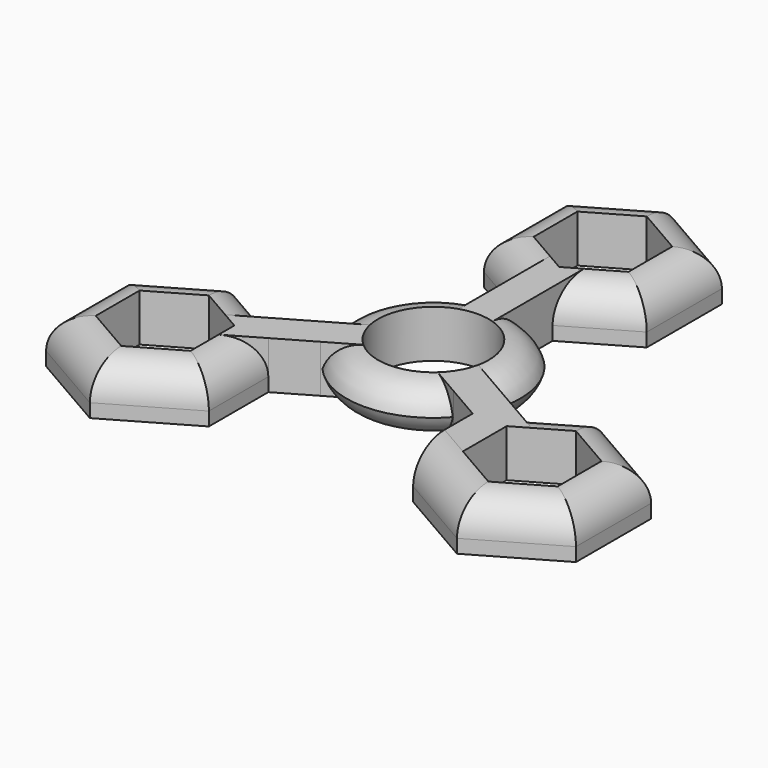
from build123d import *

# Parameters (mm, degrees)
F0_R          = 8.15
F1_DEPTH      = 7
F2_T4_DEPTH   = 35.9367513459
F2_T10_DEPTH  = 38.8235026919
F2_T16_DEPTH  = 38.8235026919
F2_T22_DEPTH  = 38.8235026919
F2_T28_DEPTH  = 38.8235026919
F2_T34_DEPTH  = 35.9367513459
F2_T40_DEPTH  = 38.8235026919
F2_T46_DEPTH  = 38.8235026919
F2_T52_DEPTH  = 38.8235026919
F2_T58_DEPTH  = 35.9367513459
F2_T64_DEPTH  = 38.8235026919
F2_T70_DEPTH  = 38.8235026919
F2_T76_DEPTH  = 38.8235026919
F2_T82_DEPTH  = 38.8235026919
F2_T88_DEPTH  = 38.8235026919
F2_T94_DEPTH  = 35.9367513459
F2_T100_DEPTH = 35.9367513459
F2_T106_ANGLE = 208.0615087698
F2_T112_ANGLE = 208.0615087698
F2_T118_ANGLE = 208.0615087698
F2_T124_ANGLE = 208.0615087698
F2_T130_ANGLE = 208.0615087698
F2_T136_ANGLE = 208.0615087698
F2_T143_DEPTH = 35.9367513459
F2_T147_DEPTH = 38.8235026919
F2_T154_DEPTH = 38.8235026919
F2_T158_DEPTH = 38.8235026919
F2_T165_DEPTH = 38.8235026919
F2_T169_DEPTH = 38.8235026919
F2_T176_DEPTH = 38.8235026919
F2_T180_DEPTH = 38.8235026919
F2_T187_DEPTH = 38.8235026919
F2_T191_DEPTH = 35.9367513459
F2_T198_DEPTH = 38.8235026919
F2_T202_DEPTH = 38.8235026919
F2_T209_DEPTH = 38.8235026919
F2_T213_DEPTH = 38.8235026919
F2_T220_DEPTH = 38.8235026919
F2_T224_DEPTH = 38.8235026919
F2_T231_DEPTH = 38.8235026919
F2_T235_DEPTH = 35.9367513459
F2_T242_DEPTH = 38.8235026919
F2_T246_DEPTH = 38.8235026919
F2_T253_DEPTH = 38.8235026919
F2_T257_DEPTH = 35.9367513459
F2_T264_DEPTH = 38.8235026919
F2_T268_DEPTH = 38.8235026919
F2_T275_DEPTH = 38.8235026919
F2_T279_DEPTH = 38.8235026919
F2_T286_DEPTH = 35.9367513459
F2_T290_DEPTH = 38.8235026919


# Not quite as in the source:
# - a fillet or chamfer that OpenCascade refuses, or shapes differently, is made with other operations: its cross-section is extruded or revolved along the edge and cut away or added


with BuildPart() as f1:
    # F0 (on Top) → F1 (new body)
    with BuildSketch(Plane.XY):
        with BuildLine():
            ThreePointArc((12.298189897, -4.2136119016), (12.8233472358, -2.1358290357), (13, 0))
            ThreePointArc((13, 0), (10.0374299499, 8.2613558209), (2.5, 12.7573508222))
            ThreePointArc((2.5, 12.7573508222), (0, 13), (-2.5, 12.7573508222))
            ThreePointArc((-2.5, 12.7573508222), (-11.2583302492, 6.5), (-12.298189897, -4.2136119016))
            ThreePointArc((-12.298189897, -4.2136119016), (-11.2583302492, -6.5), (-9.798189897, -8.5437389205))
            ThreePointArc((-9.798189897, -8.5437389205), (0, -13), (9.798189897, -8.5437389205))
            ThreePointArc((9.798189897, -8.5437389205), (11.2583302492, -6.5), (12.298189897, -4.2136119016))
        make_face()
        Circle(F0_R, mode=Mode.SUBTRACT)
        with BuildLine():
            ThreePointArc((-2.5, 12.7573508222), (0, 13), (2.5, 12.7573508222))
            Line((2.5, 12.7573508222), (2.5, 18.7963702892))
            Line((2.5, 18.7963702892), (11.9715045005, 24.2647459622))
            Line((11.9715045005, 24.2647459622), (11.9715045005, 38.0882486541))
            Line((11.9715045005, 38.0882486541), (0, 45))
            Line((0, 45), (-11.9715045005, 38.0882486541))
            Line((-11.9715045005, 38.0882486541), (-11.9715045005, 24.2647459622))
            Line((-11.9715045005, 24.2647459622), (-5.9857522502, 20.8088702892))
            Line((-5.9857522502, 20.8088702892), (-2.5, 18.7963702892))
            Line((-2.5, 18.7963702892), (-2.5, 12.7573508222))
        make_face()
        Polygon((0, 39.2264973081), (6.9715045005, 35.2014973081), (6.9715045005, 27.1514973081), (0, 23.1264973081), (-6.9715045005, 27.1514973081), (-6.9715045005, 35.2014973081), align=None, mode=Mode.SUBTRACT)
        with BuildLine():
            Line((17.5281341694, -7.2331216351), (12.298189897, -4.2136119016))
            ThreePointArc((12.298189897, -4.2136119016), (11.2583302492, -6.5), (9.798189897, -8.5437389205))
            Line((9.798189897, -8.5437389205), (15.0281341694, -11.5632486541))
            Line((15.0281341694, -11.5632486541), (15.0281341694, -22.5))
            Line((15.0281341694, -22.5), (26.9996386698, -29.4117513459))
            Line((26.9996386698, -29.4117513459), (38.9711431703, -22.5))
            Line((38.9711431703, -22.5), (38.9711431703, -8.6764973081))
            Line((38.9711431703, -8.6764973081), (26.9996386698, -1.7647459622))
            Line((26.9996386698, -1.7647459622), (21.0138864196, -5.2206216351))
            Line((21.0138864196, -5.2206216351), (17.5281341694, -7.2331216351))
        make_face()
        Polygon((33.9711431703, -19.6132486541), (26.9996386698, -23.6382486541), (20.0281341694, -19.6132486541), (20.0281341694, -11.5632486541), (26.9996386698, -7.5382486541), (33.9711431703, -11.5632486541), align=None, mode=Mode.SUBTRACT)
        with BuildLine():
            ThreePointArc((-9.798189897, -8.5437389205), (-11.2583302492, -6.5), (-12.298189897, -4.2136119016))
            Line((-12.298189897, -4.2136119016), (-17.5281341694, -7.2331216351))
            Line((-17.5281341694, -7.2331216351), (-26.9996386698, -1.7647459622))
            Line((-26.9996386698, -1.7647459622), (-38.9711431703, -8.6764973081))
            Line((-38.9711431703, -8.6764973081), (-38.9711431703, -22.5))
            Line((-38.9711431703, -22.5), (-26.9996386698, -29.4117513459))
            Line((-26.9996386698, -29.4117513459), (-15.0281341694, -22.5))
            Line((-15.0281341694, -22.5), (-15.0281341694, -15.5882486541))
            Line((-15.0281341694, -15.5882486541), (-15.0281341694, -11.5632486541))
            Line((-15.0281341694, -11.5632486541), (-9.798189897, -8.5437389205))
        make_face()
        Polygon((-33.9711431703, -19.6132486541), (-33.9711431703, -11.5632486541), (-26.9996386698, -7.5382486541), (-20.0281341694, -11.5632486541), (-20.0281341694, -19.6132486541), (-26.9996386698, -23.6382486541), align=None, mode=Mode.SUBTRACT)
    extrude(amount=F1_DEPTH)

    # F2: fillet of radius 5 on 23 edges, made by hand


with BuildPart() as f2_tool2:
    # F2_s3 → F2_t4 (new body)
    with BuildSketch(Plane(origin=(0.8112504626, -0.468375673, 0), x_dir=(0, 0, 1), z_dir=(-0.8660254038, 0.5, 0))):
        with BuildLine():
            ThreePointArc((2, -15.0281341694), (5.5355339059, -16.4926002634), (7, -20.0281341694))
            Line((7, -20.0281341694), (7.1, -20.0281341694))
            Line((7.1, -20.0281341694), (7.1, -14.9281341694))
            Line((7.1, -14.9281341694), (2, -14.9281341694))
            Line((2, -14.9281341694), (2, -15.0281341694))
        make_face()
    extrude(amount=F2_T4_DEPTH)

    split(bisect_by=Plane(origin=(-1.25, 2.1650635095, 0), x_dir=(0, 0, 1), z_dir=(-0.5, 0.8660254038, 0)), keep=Keep.TOP)

    split(bisect_by=Plane(origin=(-5.9857522502, 10.3676270189, 0), x_dir=(0, 0, 1), z_dir=(0.5, -0.8660254038, 0)), keep=Keep.TOP)


with BuildPart() as f1_1:
    add(f1.part)

    # F2_t1: cut F2_tool2
    add(f2_tool2.part, mode=Mode.SUBTRACT)


with BuildPart() as f2_tool8:
    # F2_s9 → F2_t10 (new body)
    with BuildSketch(Plane(origin=(-10.1885688723, -5.8823729811, 0), x_dir=(0, 0, 1), z_dir=(-0.8660254038, -0.5, 0))):
        with BuildLine():
            ThreePointArc((2, 11.9715045005), (5.5355339059, 10.5070384064), (7, 6.9715045005))
            Line((7, 6.9715045005), (7.1, 6.9715045005))
            Line((7.1, 6.9715045005), (7.1, 12.0715045005))
            Line((7.1, 12.0715045005), (2, 12.0715045005))
            Line((2, 12.0715045005), (2, 11.9715045005))
        make_face()
    extrude(amount=F2_T10_DEPTH)

    split(bisect_by=Plane(origin=(-7.5140670847, -13.0147459622, 0), x_dir=(0, 0, 1), z_dir=(-0.5, -0.8660254038, 0)), keep=Keep.TOP)

    split(bisect_by=Plane.YZ.offset(-38.9711431703), keep=Keep.TOP)


with BuildPart() as f1_2:
    add(f1_1.part)

    # F2_t7: cut F2_tool8
    add(f2_tool8.part, mode=Mode.SUBTRACT)


with BuildPart() as f2_tool14:
    # F2_s15 → F2_t16 (new body)
    with BuildSketch(Plane.XZ.offset(-3.8235026919)):
        with BuildLine():
            ThreePointArc((-38.9711431703, 2), (-37.5066770762, 5.5355339059), (-33.9711431703, 7))
            Line((-33.9711431703, 7), (-33.9711431703, 7.1))
            Line((-33.9711431703, 7.1), (-39.0711431703, 7.1))
            Line((-39.0711431703, 7.1), (-39.0711431703, 2))
            Line((-39.0711431703, 2), (-38.9711431703, 2))
        make_face()
    extrude(amount=F2_T16_DEPTH)

    split(bisect_by=Plane(origin=(-5.9857522502, 10.3676270189, 0), x_dir=(0, 0, 1), z_dir=(0.5, -0.8660254038, 0)), keep=Keep.TOP)

    split(bisect_by=Plane(origin=(-19.4855715851, -33.75, 0), x_dir=(0, 0, 1), z_dir=(0.5, 0.8660254038, 0)), keep=Keep.TOP)


with BuildPart() as f1_3:
    add(f1_2.part)

    # F2_t13: cut F2_tool14
    add(f2_tool14.part, mode=Mode.SUBTRACT)


with BuildPart() as f2_tool20:
    # F2_s21 → F2_t22 (new body)
    with BuildSketch(Plane(origin=(-30.3108891325, 17.5, 0), x_dir=(0, 0, 1), z_dir=(0.8660254038, -0.5, 0))):
        with BuildLine():
            ThreePointArc((2, 38.9711431703), (5.5355339059, 37.5066770762), (7, 33.9711431703))
            Line((7, 33.9711431703), (7.1, 33.9711431703))
            Line((7.1, 33.9711431703), (7.1, 39.0711431703))
            Line((7.1, 39.0711431703), (2, 39.0711431703))
            Line((2, 39.0711431703), (2, 38.9711431703))
        make_face()
    extrude(amount=F2_T22_DEPTH)

    split(bisect_by=Plane.YZ.offset(-38.9711431703), keep=Keep.TOP)

    split(bisect_by=Plane(origin=(5.9857522502, -10.3676270189, 0), x_dir=(0, 0, 1), z_dir=(-0.5, 0.8660254038, 0)), keep=Keep.TOP)


with BuildPart() as f1_4:
    add(f1_3.part)

    # F2_t19: cut F2_tool20
    add(f2_tool20.part, mode=Mode.SUBTRACT)


with BuildPart() as f2_tool26:
    # F2_s27 → F2_t28 (new body)
    with BuildSketch(Plane(origin=(-43.8107084674, -25.294124327, 0), x_dir=(0, 0, 1), z_dir=(0.8660254038, 0.5, 0))):
        with BuildLine():
            ThreePointArc((2, 11.9715045005), (5.5355339059, 10.5070384064), (7, 6.9715045005))
            Line((7, 6.9715045005), (7.1, 6.9715045005))
            Line((7.1, 6.9715045005), (7.1, 12.0715045005))
            Line((7.1, 12.0715045005), (2, 12.0715045005))
            Line((2, 12.0715045005), (2, 11.9715045005))
        make_face()
    extrude(amount=F2_T28_DEPTH)

    split(bisect_by=Plane(origin=(-19.4855715851, -33.75, 0), x_dir=(0, 0, 1), z_dir=(0.5, 0.8660254038, 0)), keep=Keep.TOP)

    split(bisect_by=Plane.YZ.offset(-15.0281341694), keep=Keep.BOTTOM)


with BuildPart() as f1_5:
    add(f1_4.part)

    # F2_t25: cut F2_tool26
    add(f2_tool26.part, mode=Mode.SUBTRACT)


with BuildPart() as f2_tool32:
    # F2_s33 → F2_t34 (new body)
    with BuildSketch(Plane.XZ.offset(35)):
        with BuildLine():
            ThreePointArc((-15.0281341694, 2), (-16.4926002634, 5.5355339059), (-20.0281341694, 7))
            Line((-20.0281341694, 7), (-20.0281341694, 7.1))
            Line((-20.0281341694, 7.1), (-14.9281341694, 7.1))
            Line((-14.9281341694, 7.1), (-14.9281341694, 2))
            Line((-14.9281341694, 2), (-15.0281341694, 2))
        make_face()
    extrude(amount=-F2_T34_DEPTH)

    split(bisect_by=Plane(origin=(5.9857522502, -10.3676270189, 0), x_dir=(0, 0, 1), z_dir=(-0.5, 0.8660254038, 0)), keep=Keep.TOP)

    split(bisect_by=Plane(origin=(1.25, -2.1650635095, 0), x_dir=(0, 0, 1), z_dir=(0.5, -0.8660254038, 0)), keep=Keep.TOP)


with BuildPart() as f1_6:
    add(f1_5.part)

    # F2_t31: cut F2_tool32
    add(f2_tool32.part, mode=Mode.SUBTRACT)


with BuildPart() as f2_tool38:
    # F2_s39 → F2_t40 (new body)
    with BuildSketch(Plane(origin=(-3.3112504626, -1.9117513459, 0), x_dir=(0, 0, 1), z_dir=(0.8660254038, 0.5, 0))):
        with BuildLine():
            ThreePointArc((2, 38.9711431703), (5.5355339059, 37.5066770762), (7, 33.9711431703))
            Line((7, 33.9711431703), (7.1, 33.9711431703))
            Line((7.1, 33.9711431703), (7.1, 39.0711431703))
            Line((7.1, 39.0711431703), (2, 39.0711431703))
            Line((2, 39.0711431703), (2, 38.9711431703))
        make_face()
    extrude(amount=F2_T40_DEPTH)

    split(bisect_by=Plane(origin=(-5.9857522502, -10.3676270189, 0), x_dir=(0, 0, 1), z_dir=(0.5, 0.8660254038, 0)), keep=Keep.TOP)

    split(bisect_by=Plane.YZ.offset(38.9711431703), keep=Keep.BOTTOM)


with BuildPart() as f1_7:
    add(f1_6.part)

    # F2_t37: cut F2_tool38
    add(f2_tool38.part, mode=Mode.SUBTRACT)


with BuildPart() as f2_tool44:
    # F2_s45 → F2_t46 (new body)
    with BuildSketch(Plane.XZ.offset(35)):
        with BuildLine():
            ThreePointArc((38.9711431703, 2), (37.5066770762, 5.5355339059), (33.9711431703, 7))
            Line((33.9711431703, 7), (33.9711431703, 7.1))
            Line((33.9711431703, 7.1), (39.0711431703, 7.1))
            Line((39.0711431703, 7.1), (39.0711431703, 2))
            Line((39.0711431703, 2), (38.9711431703, 2))
        make_face()
    extrude(amount=-F2_T46_DEPTH)

    split(bisect_by=Plane(origin=(19.4855715851, -33.75, 0), x_dir=(0, 0, 1), z_dir=(-0.5, 0.8660254038, 0)), keep=Keep.TOP)

    split(bisect_by=Plane(origin=(5.9857522502, 10.3676270189, 0), x_dir=(0, 0, 1), z_dir=(-0.5, -0.8660254038, 0)), keep=Keep.TOP)


with BuildPart() as f1_8:
    add(f1_7.part)

    # F2_t43: cut F2_tool44
    add(f2_tool44.part, mode=Mode.SUBTRACT)


with BuildPart() as f2_tool50:
    # F2_s51 → F2_t52 (new body)
    with BuildSketch(Plane(origin=(43.8107084674, -25.294124327, 0), x_dir=(0, 0, 1), z_dir=(-0.8660254038, 0.5, 0))):
        with BuildLine():
            ThreePointArc((2, 11.9715045005), (5.5355339059, 10.5070384064), (7, 6.9715045005))
            Line((7, 6.9715045005), (7.1, 6.9715045005))
            Line((7.1, 6.9715045005), (7.1, 12.0715045005))
            Line((7.1, 12.0715045005), (2, 12.0715045005))
            Line((2, 12.0715045005), (2, 11.9715045005))
        make_face()
    extrude(amount=F2_T52_DEPTH)

    split(bisect_by=Plane.YZ.offset(38.9711431703), keep=Keep.BOTTOM)

    split(bisect_by=Plane(origin=(7.5140670847, -13.0147459622, 0), x_dir=(0, 0, 1), z_dir=(0.5, -0.8660254038, 0)), keep=Keep.TOP)


with BuildPart() as f1_9:
    add(f1_8.part)

    # F2_t49: cut F2_tool50
    add(f2_tool50.part, mode=Mode.SUBTRACT)


with BuildPart() as f2_tool56:
    # F2_s57 → F2_t58 (new body)
    with BuildSketch(Plane(origin=(30.3108891325, 17.5, 0), x_dir=(0, 0, 1), z_dir=(-0.8660254038, -0.5, 0))):
        with BuildLine():
            ThreePointArc((2, -15.0281341694), (5.5355339059, -16.4926002634), (7, -20.0281341694))
            Line((7, -20.0281341694), (7.1, -20.0281341694))
            Line((7.1, -20.0281341694), (7.1, -14.9281341694))
            Line((7.1, -14.9281341694), (2, -14.9281341694))
            Line((2, -14.9281341694), (2, -15.0281341694))
        make_face()
    extrude(amount=F2_T58_DEPTH)

    split(bisect_by=Plane(origin=(5.9857522502, 10.3676270189, 0), x_dir=(0, 0, 1), z_dir=(-0.5, -0.8660254038, 0)), keep=Keep.TOP)

    split(bisect_by=Plane(origin=(1.25, 2.1650635095, 0), x_dir=(0, 0, 1), z_dir=(0.5, 0.8660254038, 0)), keep=Keep.TOP)


with BuildPart() as f1_10:
    add(f1_9.part)

    # F2_t55: cut F2_tool56
    add(f2_tool56.part, mode=Mode.SUBTRACT)


with BuildPart() as f2_tool62:
    # F2_s63 → F2_t64 (new body)
    with BuildSketch(Plane(origin=(10.1885688723, -5.8823729811, 0), x_dir=(0, 0, 1), z_dir=(0.8660254038, -0.5, 0))):
        with BuildLine():
            ThreePointArc((2, 11.9715045005), (5.5355339059, 10.5070384064), (7, 6.9715045005))
            Line((7, 6.9715045005), (7.1, 6.9715045005))
            Line((7.1, 6.9715045005), (7.1, 12.0715045005))
            Line((7.1, 12.0715045005), (2, 12.0715045005))
            Line((2, 12.0715045005), (2, 11.9715045005))
        make_face()
    extrude(amount=F2_T64_DEPTH)

    split(bisect_by=Plane.YZ.offset(15.0281341694), keep=Keep.TOP)

    split(bisect_by=Plane(origin=(19.4855715851, -33.75, 0), x_dir=(0, 0, 1), z_dir=(-0.5, 0.8660254038, 0)), keep=Keep.TOP)


with BuildPart() as f1_11:
    add(f1_10.part)

    # F2_t61: cut F2_tool62
    add(f2_tool62.part, mode=Mode.SUBTRACT)


with BuildPart() as f2_tool68:
    # F2_s69 → F2_t70 (new body)
    with BuildSketch(Plane.XZ.offset(-50.5882486541)):
        with BuildLine():
            ThreePointArc((-11.9715045005, 2), (-10.5070384064, 5.5355339059), (-6.9715045005, 7))
            Line((-6.9715045005, 7), (-6.9715045005, 7.1))
            Line((-6.9715045005, 7.1), (-12.0715045005, 7.1))
            Line((-12.0715045005, 7.1), (-12.0715045005, 2))
            Line((-12.0715045005, 2), (-11.9715045005, 2))
        make_face()
    extrude(amount=F2_T70_DEPTH)

    split(bisect_by=Plane(origin=(-19.4855715851, 33.75, 0), x_dir=(0, 0, 1), z_dir=(0.5, -0.8660254038, 0)), keep=Keep.TOP)

    split(bisect_by=Plane(origin=(7.5140670847, 13.0147459622, 0), x_dir=(0, 0, 1), z_dir=(0.5, 0.8660254038, 0)), keep=Keep.TOP)


with BuildPart() as f1_12:
    add(f1_11.part)

    # F2_t67: cut F2_tool68
    add(f2_tool68.part, mode=Mode.SUBTRACT)


with BuildPart() as f2_tool74:
    # F2_s75 → F2_t76 (new body)
    with BuildSketch(Plane(origin=(30.3108891325, 17.5, 0), x_dir=(0, 0, 1), z_dir=(-0.8660254038, -0.5, 0))):
        with BuildLine():
            ThreePointArc((2, 38.9711431703), (5.5355339059, 37.5066770762), (7, 33.9711431703))
            Line((7, 33.9711431703), (7.1, 33.9711431703))
            Line((7.1, 33.9711431703), (7.1, 39.0711431703))
            Line((7.1, 39.0711431703), (2, 39.0711431703))
            Line((2, 39.0711431703), (2, 38.9711431703))
        make_face()
    extrude(amount=F2_T76_DEPTH)

    split(bisect_by=Plane(origin=(19.4855715851, 33.75, 0), x_dir=(0, 0, 1), z_dir=(-0.5, -0.8660254038, 0)), keep=Keep.TOP)

    split(bisect_by=Plane.YZ.offset(-11.9715045005), keep=Keep.TOP)


with BuildPart() as f1_13:
    add(f1_12.part)

    # F2_t73: cut F2_tool74
    add(f2_tool74.part, mode=Mode.SUBTRACT)


with BuildPart() as f2_tool80:
    # F2_s81 → F2_t82 (new body)
    with BuildSketch(Plane(origin=(3.3112504626, -1.9117513459, 0), x_dir=(0, 0, 1), z_dir=(-0.8660254038, 0.5, 0))):
        with BuildLine():
            ThreePointArc((2, 38.9711431703), (5.5355339059, 37.5066770762), (7, 33.9711431703))
            Line((7, 33.9711431703), (7.1, 33.9711431703))
            Line((7.1, 33.9711431703), (7.1, 39.0711431703))
            Line((7.1, 39.0711431703), (2, 39.0711431703))
            Line((2, 39.0711431703), (2, 38.9711431703))
        make_face()
    extrude(amount=F2_T82_DEPTH)

    split(bisect_by=Plane.YZ.offset(11.9715045005), keep=Keep.BOTTOM)

    split(bisect_by=Plane(origin=(-19.4855715851, 33.75, 0), x_dir=(0, 0, 1), z_dir=(0.5, -0.8660254038, 0)), keep=Keep.TOP)


with BuildPart() as f1_14:
    add(f1_13.part)

    # F2_t79: cut F2_tool80
    add(f2_tool80.part, mode=Mode.SUBTRACT)


with BuildPart() as f2_tool86:
    # F2_s87 → F2_t88 (new body)
    with BuildSketch(Plane.XZ.offset(-11.7647459622)):
        with BuildLine():
            ThreePointArc((11.9715045005, 2), (10.5070384064, 5.5355339059), (6.9715045005, 7))
            Line((6.9715045005, 7), (6.9715045005, 7.1))
            Line((6.9715045005, 7.1), (12.0715045005, 7.1))
            Line((12.0715045005, 7.1), (12.0715045005, 2))
            Line((12.0715045005, 2), (11.9715045005, 2))
        make_face()
    extrude(amount=-F2_T88_DEPTH)

    split(bisect_by=Plane(origin=(-7.5140670847, 13.0147459622, 0), x_dir=(0, 0, 1), z_dir=(-0.5, 0.8660254038, 0)), keep=Keep.TOP)

    split(bisect_by=Plane(origin=(19.4855715851, 33.75, 0), x_dir=(0, 0, 1), z_dir=(-0.5, -0.8660254038, 0)), keep=Keep.TOP)


with BuildPart() as f1_15:
    add(f1_14.part)

    # F2_t85: cut F2_tool86
    add(f2_tool86.part, mode=Mode.SUBTRACT)


with BuildPart() as f2_tool92:
    # F2_s93 → F2_t94 (new body)
    with BuildSketch(Plane(origin=(-30.3108891325, 17.5, 0), x_dir=(0, 0, 1), z_dir=(0.8660254038, -0.5, 0))):
        with BuildLine():
            ThreePointArc((2, -15.0281341694), (5.5355339059, -16.4926002634), (7, -20.0281341694))
            Line((7, -20.0281341694), (7.1, -20.0281341694))
            Line((7.1, -20.0281341694), (7.1, -14.9281341694))
            Line((7.1, -14.9281341694), (2, -14.9281341694))
            Line((2, -14.9281341694), (2, -15.0281341694))
        make_face()
    extrude(amount=F2_T94_DEPTH)

    split(bisect_by=Plane.YZ.offset(-11.9715045005), keep=Keep.TOP)

    split(bisect_by=Plane.YZ.offset(-2.5), keep=Keep.BOTTOM)


with BuildPart() as f1_16:
    add(f1_15.part)

    # F2_t91: cut F2_tool92
    add(f2_tool92.part, mode=Mode.SUBTRACT)


with BuildPart() as f2_tool98:
    # F2_s99 → F2_t100 (new body)
    with BuildSketch(Plane(origin=(-0.8112504626, -0.468375673, 0), x_dir=(0, 0, 1), z_dir=(0.8660254038, 0.5, 0))):
        with BuildLine():
            ThreePointArc((2, -15.0281341694), (5.5355339059, -16.4926002634), (7, -20.0281341694))
            Line((7, -20.0281341694), (7.1, -20.0281341694))
            Line((7.1, -20.0281341694), (7.1, -14.9281341694))
            Line((7.1, -14.9281341694), (2, -14.9281341694))
            Line((2, -14.9281341694), (2, -15.0281341694))
        make_face()
    extrude(amount=F2_T100_DEPTH)

    split(bisect_by=Plane.YZ.offset(2.5), keep=Keep.TOP)

    split(bisect_by=Plane.YZ.offset(11.9715045005), keep=Keep.BOTTOM)


with BuildPart() as f1_17:
    add(f1_16.part)

    # F2_t97: cut F2_tool98
    add(f2_tool98.part, mode=Mode.SUBTRACT)


with BuildPart() as f2_tool104:
    # F2_s105 → F2_t106 (revolve)
    with BuildSketch(Plane(origin=(0, 0, 0), x_dir=(0, 0, 1), z_dir=(0.7189668282, -0.695044387, 0))):
        with BuildLine():
            ThreePointArc((2, -13), (5.5355339059, -11.5355339059), (7, -8))
            Line((7, -8), (7.1, -8))
            Line((7.1, -8), (7.1, -13.1))
            Line((7.1, -13.1), (2, -13.1))
            Line((2, -13.1), (2, -13))
        make_face()
    revolve(axis=Axis((0, 0, 7), (0, 0, 1)), revolution_arc=F2_T106_ANGLE)

    split(bisect_by=Plane.YZ.offset(-2.5), keep=Keep.BOTTOM)

    split(bisect_by=Plane(origin=(-1.25, 2.1650635095, 0), x_dir=(0, 0, 1), z_dir=(-0.5, 0.8660254038, 0)), keep=Keep.TOP)


with BuildPart() as f1_18:
    add(f1_17.part)

    # F2_t103: cut F2_tool104
    add(f2_tool104.part, mode=Mode.SUBTRACT)


with BuildPart() as f2_tool110:
    # F2_s111 → F2_t112 (revolve)
    with BuildSketch(Plane(origin=(0, 0, 0), x_dir=(0, 0, 1), z_dir=(-0.96140951, -0.2751213442, 0))):
        with BuildLine():
            ThreePointArc((2, -13), (5.5355339059, -11.5355339059), (7, -8))
            Line((7, -8), (7.1, -8))
            Line((7.1, -8), (7.1, -13.1))
            Line((7.1, -13.1), (2, -13.1))
            Line((2, -13.1), (2, -13))
        make_face()
    revolve(axis=Axis((0, 0, 7), (0, 0, 1)), revolution_arc=F2_T112_ANGLE)

    split(bisect_by=Plane.YZ.offset(2.5), keep=Keep.TOP)

    split(bisect_by=Plane(origin=(1.25, 2.1650635095, 0), x_dir=(0, 0, 1), z_dir=(0.5, 0.8660254038, 0)), keep=Keep.TOP)


with BuildPart() as f1_19:
    add(f1_18.part)

    # F2_t109: cut F2_tool110
    add(f2_tool110.part, mode=Mode.SUBTRACT)


with BuildPart() as f2_tool116:
    # F2_s117 → F2_t118 (revolve)
    with BuildSketch(Plane(origin=(0, 0, 0), x_dir=(0, 0, 1), z_dir=(0.2424426818, 0.9701657312, 0))):
        with BuildLine():
            ThreePointArc((2, -13), (5.5355339059, -11.5355339059), (7, -8))
            Line((7, -8), (7.1, -8))
            Line((7.1, -8), (7.1, -13.1))
            Line((7.1, -13.1), (2, -13.1))
            Line((2, -13.1), (2, -13))
        make_face()
    revolve(axis=Axis((0, 0, 7), (0, 0, 1)), revolution_arc=F2_T118_ANGLE)

    split(bisect_by=Plane(origin=(1.25, -2.1650635095, 0), x_dir=(0, 0, 1), z_dir=(0.5, -0.8660254038, 0)), keep=Keep.TOP)

    split(bisect_by=Plane(origin=(-1.25, -2.1650635095, 0), x_dir=(0, 0, 1), z_dir=(-0.5, -0.8660254038, 0)), keep=Keep.TOP)


with BuildPart() as f1_20:
    add(f1_19.part)

    # F2_t115: cut F2_tool116
    add(f2_tool116.part, mode=Mode.SUBTRACT)


with BuildPart() as f2_tool122:
    # F2_s123 → F2_t124 (revolve)
    with BuildSketch(Plane(origin=(0, 0, 0), x_dir=(0, 0, 1), z_dir=(0.2424426818, 0.9701657312, 0))):
        with BuildLine():
            ThreePointArc((5, -13), (1.4644660941, -11.5355339059), (0, -8))
            Line((0, -8), (-0.1, -8))
            Line((-0.1, -8), (-0.1, -13.1))
            Line((-0.1, -13.1), (5, -13.1))
            Line((5, -13.1), (5, -13))
        make_face()
    revolve(axis=Axis((0, 0, 0), (0, 0, 1)), revolution_arc=F2_T124_ANGLE)

    split(bisect_by=Plane(origin=(1.25, -2.1650635095, 0), x_dir=(0, 0, 1), z_dir=(0.5, -0.8660254038, 0)), keep=Keep.TOP)

    split(bisect_by=Plane(origin=(-1.25, -2.1650635095, 0), x_dir=(0, 0, 1), z_dir=(-0.5, -0.8660254038, 0)), keep=Keep.TOP)


with BuildPart() as f1_21:
    add(f1_20.part)

    # F2_t121: cut F2_tool122
    add(f2_tool122.part, mode=Mode.SUBTRACT)


with BuildPart() as f2_tool128:
    # F2_s129 → F2_t130 (revolve)
    with BuildSketch(Plane(origin=(0, 0, 0), x_dir=(0, 0, 1), z_dir=(-0.96140951, -0.2751213442, 0))):
        with BuildLine():
            ThreePointArc((5, -13), (1.4644660941, -11.5355339059), (0, -8))
            Line((0, -8), (-0.1, -8))
            Line((-0.1, -8), (-0.1, -13.1))
            Line((-0.1, -13.1), (5, -13.1))
            Line((5, -13.1), (5, -13))
        make_face()
    revolve(axis=Axis((0, 0, 0), (0, 0, 1)), revolution_arc=F2_T130_ANGLE)

    split(bisect_by=Plane.YZ.offset(2.5), keep=Keep.TOP)

    split(bisect_by=Plane(origin=(1.25, 2.1650635095, 0), x_dir=(0, 0, 1), z_dir=(0.5, 0.8660254038, 0)), keep=Keep.TOP)


with BuildPart() as f1_22:
    add(f1_21.part)

    # F2_t127: cut F2_tool128
    add(f2_tool128.part, mode=Mode.SUBTRACT)


with BuildPart() as f2_tool134:
    # F2_s135 → F2_t136 (revolve)
    with BuildSketch(Plane(origin=(0, 0, 0), x_dir=(0, 0, 1), z_dir=(0.7189668282, -0.695044387, 0))):
        with BuildLine():
            ThreePointArc((5, -13), (1.4644660941, -11.5355339059), (0, -8))
            Line((0, -8), (-0.1, -8))
            Line((-0.1, -8), (-0.1, -13.1))
            Line((-0.1, -13.1), (5, -13.1))
            Line((5, -13.1), (5, -13))
        make_face()
    revolve(axis=Axis((0, 0, 0), (0, 0, 1)), revolution_arc=F2_T136_ANGLE)

    split(bisect_by=Plane.YZ.offset(-2.5), keep=Keep.BOTTOM)

    split(bisect_by=Plane(origin=(-1.25, 2.1650635095, 0), x_dir=(0, 0, 1), z_dir=(-0.5, 0.8660254038, 0)), keep=Keep.TOP)


with BuildPart() as f1_23:
    add(f1_22.part)

    # F2_t133: cut F2_tool134
    add(f2_tool134.part, mode=Mode.SUBTRACT)


with BuildPart() as f2_tool141:
    # F2_s142 → F2_t143 (new body)
    with BuildSketch(Plane(origin=(0.8112504626, -0.468375673, 0), x_dir=(0, 0, 1), z_dir=(-0.8660254038, 0.5, 0))):
        with BuildLine():
            ThreePointArc((2, -15.0281341694), (5.5355339059, -16.4926002634), (7, -20.0281341694))
            Line((7, -20.0281341694), (7.1, -20.0281341694))
            Line((7.1, -20.0281341694), (7.1, -14.9281341694))
            Line((7.1, -14.9281341694), (2, -14.9281341694))
            Line((2, -14.9281341694), (2, -15.0281341694))
        make_face()
    extrude(amount=F2_T143_DEPTH)

    split(bisect_by=Plane(origin=(-5.9857522502, 10.3676270189, 0), x_dir=(0, 0, 1), z_dir=(-0.5, 0.8660254038, 0)), keep=Keep.TOP)


with BuildPart() as f2_tool145:
    # F2_s146 → F2_t147 (new body)
    with BuildSketch(Plane(origin=(-10.1885688723, -5.8823729811, 0), x_dir=(0, 0, 1), z_dir=(-0.8660254038, -0.5, 0))):
        with BuildLine():
            ThreePointArc((2, 11.9715045005), (5.5355339059, 10.5070384064), (7, 6.9715045005))
            Line((7, 6.9715045005), (7.1, 6.9715045005))
            Line((7.1, 6.9715045005), (7.1, 12.0715045005))
            Line((7.1, 12.0715045005), (2, 12.0715045005))
            Line((2, 12.0715045005), (2, 11.9715045005))
        make_face()
    extrude(amount=F2_T147_DEPTH)

    split(bisect_by=Plane(origin=(-7.5140670847, -13.0147459622, 0), x_dir=(0, 0, 1), z_dir=(0.5, 0.8660254038, 0)), keep=Keep.TOP)


with BuildPart() as f2_tool141_1:
    add(f2_tool141.part)

    # F2_t149: intersect F2_tool145
    add(f2_tool145.part, mode=Mode.INTERSECT)


with BuildPart() as f1_24:
    add(f1_23.part)

    # F2_t139: cut F2_tool141
    add(f2_tool141_1.part, mode=Mode.SUBTRACT)


with BuildPart() as f2_tool152:
    # F2_s153 → F2_t154 (new body)
    with BuildSketch(Plane(origin=(-10.1885688723, -5.8823729811, 0), x_dir=(0, 0, 1), z_dir=(-0.8660254038, -0.5, 0))):
        with BuildLine():
            ThreePointArc((2, 11.9715045005), (5.5355339059, 10.5070384064), (7, 6.9715045005))
            Line((7, 6.9715045005), (7.1, 6.9715045005))
            Line((7.1, 6.9715045005), (7.1, 12.0715045005))
            Line((7.1, 12.0715045005), (2, 12.0715045005))
            Line((2, 12.0715045005), (2, 11.9715045005))
        make_face()
    extrude(amount=F2_T154_DEPTH)

    split(bisect_by=Plane.YZ.offset(-38.9711431703), keep=Keep.BOTTOM)


with BuildPart() as f2_tool156:
    # F2_s157 → F2_t158 (new body)
    with BuildSketch(Plane.XZ.offset(-3.8235026919)):
        with BuildLine():
            ThreePointArc((-38.9711431703, 2), (-37.5066770762, 5.5355339059), (-33.9711431703, 7))
            Line((-33.9711431703, 7), (-33.9711431703, 7.1))
            Line((-33.9711431703, 7.1), (-39.0711431703, 7.1))
            Line((-39.0711431703, 7.1), (-39.0711431703, 2))
            Line((-39.0711431703, 2), (-38.9711431703, 2))
        make_face()
    extrude(amount=F2_T158_DEPTH)

    split(bisect_by=Plane(origin=(-5.9857522502, 10.3676270189, 0), x_dir=(0, 0, 1), z_dir=(-0.5, 0.8660254038, 0)), keep=Keep.TOP)


with BuildPart() as f2_tool152_1:
    add(f2_tool152.part)

    # F2_t160: intersect F2_tool156
    add(f2_tool156.part, mode=Mode.INTERSECT)


with BuildPart() as f1_25:
    add(f1_24.part)

    # F2_t150: cut F2_tool152
    add(f2_tool152_1.part, mode=Mode.SUBTRACT)


with BuildPart() as f2_tool163:
    # F2_s164 → F2_t165 (new body)
    with BuildSketch(Plane.XZ.offset(-3.8235026919)):
        with BuildLine():
            ThreePointArc((-38.9711431703, 2), (-37.5066770762, 5.5355339059), (-33.9711431703, 7))
            Line((-33.9711431703, 7), (-33.9711431703, 7.1))
            Line((-33.9711431703, 7.1), (-39.0711431703, 7.1))
            Line((-39.0711431703, 7.1), (-39.0711431703, 2))
            Line((-39.0711431703, 2), (-38.9711431703, 2))
        make_face()
    extrude(amount=F2_T165_DEPTH)

    split(bisect_by=Plane(origin=(-19.4855715851, -33.75, 0), x_dir=(0, 0, 1), z_dir=(-0.5, -0.8660254038, 0)), keep=Keep.TOP)


with BuildPart() as f2_tool167:
    # F2_s168 → F2_t169 (new body)
    with BuildSketch(Plane(origin=(-30.3108891325, 17.5, 0), x_dir=(0, 0, 1), z_dir=(0.8660254038, -0.5, 0))):
        with BuildLine():
            ThreePointArc((2, 38.9711431703), (5.5355339059, 37.5066770762), (7, 33.9711431703))
            Line((7, 33.9711431703), (7.1, 33.9711431703))
            Line((7.1, 33.9711431703), (7.1, 39.0711431703))
            Line((7.1, 39.0711431703), (2, 39.0711431703))
            Line((2, 39.0711431703), (2, 38.9711431703))
        make_face()
    extrude(amount=F2_T169_DEPTH)

    split(bisect_by=Plane.YZ.offset(-38.9711431703), keep=Keep.BOTTOM)


with BuildPart() as f2_tool163_1:
    add(f2_tool163.part)

    # F2_t171: intersect F2_tool167
    add(f2_tool167.part, mode=Mode.INTERSECT)


with BuildPart() as f1_26:
    add(f1_25.part)

    # F2_t161: cut F2_tool163
    add(f2_tool163_1.part, mode=Mode.SUBTRACT)


with BuildPart() as f2_tool174:
    # F2_s175 → F2_t176 (new body)
    with BuildSketch(Plane(origin=(-30.3108891325, 17.5, 0), x_dir=(0, 0, 1), z_dir=(0.8660254038, -0.5, 0))):
        with BuildLine():
            ThreePointArc((2, 38.9711431703), (5.5355339059, 37.5066770762), (7, 33.9711431703))
            Line((7, 33.9711431703), (7.1, 33.9711431703))
            Line((7.1, 33.9711431703), (7.1, 39.0711431703))
            Line((7.1, 39.0711431703), (2, 39.0711431703))
            Line((2, 39.0711431703), (2, 38.9711431703))
        make_face()
    extrude(amount=F2_T176_DEPTH)

    split(bisect_by=Plane(origin=(5.9857522502, -10.3676270189, 0), x_dir=(0, 0, 1), z_dir=(0.5, -0.8660254038, 0)), keep=Keep.TOP)


with BuildPart() as f2_tool178:
    # F2_s179 → F2_t180 (new body)
    with BuildSketch(Plane(origin=(-43.8107084674, -25.294124327, 0), x_dir=(0, 0, 1), z_dir=(0.8660254038, 0.5, 0))):
        with BuildLine():
            ThreePointArc((2, 11.9715045005), (5.5355339059, 10.5070384064), (7, 6.9715045005))
            Line((7, 6.9715045005), (7.1, 6.9715045005))
            Line((7.1, 6.9715045005), (7.1, 12.0715045005))
            Line((7.1, 12.0715045005), (2, 12.0715045005))
            Line((2, 12.0715045005), (2, 11.9715045005))
        make_face()
    extrude(amount=F2_T180_DEPTH)

    split(bisect_by=Plane(origin=(-19.4855715851, -33.75, 0), x_dir=(0, 0, 1), z_dir=(-0.5, -0.8660254038, 0)), keep=Keep.TOP)


with BuildPart() as f2_tool174_1:
    add(f2_tool174.part)

    # F2_t182: intersect F2_tool178
    add(f2_tool178.part, mode=Mode.INTERSECT)


with BuildPart() as f1_27:
    add(f1_26.part)

    # F2_t172: cut F2_tool174
    add(f2_tool174_1.part, mode=Mode.SUBTRACT)


with BuildPart() as f2_tool185:
    # F2_s186 → F2_t187 (new body)
    with BuildSketch(Plane(origin=(-43.8107084674, -25.294124327, 0), x_dir=(0, 0, 1), z_dir=(0.8660254038, 0.5, 0))):
        with BuildLine():
            ThreePointArc((2, 11.9715045005), (5.5355339059, 10.5070384064), (7, 6.9715045005))
            Line((7, 6.9715045005), (7.1, 6.9715045005))
            Line((7.1, 6.9715045005), (7.1, 12.0715045005))
            Line((7.1, 12.0715045005), (2, 12.0715045005))
            Line((2, 12.0715045005), (2, 11.9715045005))
        make_face()
    extrude(amount=F2_T187_DEPTH)

    split(bisect_by=Plane.YZ.offset(-15.0281341694), keep=Keep.TOP)


with BuildPart() as f2_tool189:
    # F2_s190 → F2_t191 (new body)
    with BuildSketch(Plane.XZ.offset(35)):
        with BuildLine():
            ThreePointArc((-15.0281341694, 2), (-16.4926002634, 5.5355339059), (-20.0281341694, 7))
            Line((-20.0281341694, 7), (-20.0281341694, 7.1))
            Line((-20.0281341694, 7.1), (-14.9281341694, 7.1))
            Line((-14.9281341694, 7.1), (-14.9281341694, 2))
            Line((-14.9281341694, 2), (-15.0281341694, 2))
        make_face()
    extrude(amount=-F2_T191_DEPTH)

    split(bisect_by=Plane(origin=(5.9857522502, -10.3676270189, 0), x_dir=(0, 0, 1), z_dir=(0.5, -0.8660254038, 0)), keep=Keep.TOP)


with BuildPart() as f2_tool185_1:
    add(f2_tool185.part)

    # F2_t193: intersect F2_tool189
    add(f2_tool189.part, mode=Mode.INTERSECT)


with BuildPart() as f1_28:
    add(f1_27.part)

    # F2_t183: cut F2_tool185
    add(f2_tool185_1.part, mode=Mode.SUBTRACT)


with BuildPart() as f2_tool196:
    # F2_s197 → F2_t198 (new body)
    with BuildSketch(Plane(origin=(10.1885688723, -5.8823729811, 0), x_dir=(0, 0, 1), z_dir=(0.8660254038, -0.5, 0))):
        with BuildLine():
            ThreePointArc((2, 11.9715045005), (5.5355339059, 10.5070384064), (7, 6.9715045005))
            Line((7, 6.9715045005), (7.1, 6.9715045005))
            Line((7.1, 6.9715045005), (7.1, 12.0715045005))
            Line((7.1, 12.0715045005), (2, 12.0715045005))
            Line((2, 12.0715045005), (2, 11.9715045005))
        make_face()
    extrude(amount=F2_T198_DEPTH)

    split(bisect_by=Plane(origin=(19.4855715851, -33.75, 0), x_dir=(0, 0, 1), z_dir=(0.5, -0.8660254038, 0)), keep=Keep.TOP)


with BuildPart() as f2_tool200:
    # F2_s201 → F2_t202 (new body)
    with BuildSketch(Plane(origin=(-3.3112504626, -1.9117513459, 0), x_dir=(0, 0, 1), z_dir=(0.8660254038, 0.5, 0))):
        with BuildLine():
            ThreePointArc((2, 38.9711431703), (5.5355339059, 37.5066770762), (7, 33.9711431703))
            Line((7, 33.9711431703), (7.1, 33.9711431703))
            Line((7.1, 33.9711431703), (7.1, 39.0711431703))
            Line((7.1, 39.0711431703), (2, 39.0711431703))
            Line((2, 39.0711431703), (2, 38.9711431703))
        make_face()
    extrude(amount=F2_T202_DEPTH)

    split(bisect_by=Plane(origin=(-5.9857522502, -10.3676270189, 0), x_dir=(0, 0, 1), z_dir=(-0.5, -0.8660254038, 0)), keep=Keep.TOP)


with BuildPart() as f2_tool196_1:
    add(f2_tool196.part)

    # F2_t204: intersect F2_tool200
    add(f2_tool200.part, mode=Mode.INTERSECT)


with BuildPart() as f1_29:
    add(f1_28.part)

    # F2_t194: cut F2_tool196
    add(f2_tool196_1.part, mode=Mode.SUBTRACT)


with BuildPart() as f2_tool207:
    # F2_s208 → F2_t209 (new body)
    with BuildSketch(Plane(origin=(-3.3112504626, -1.9117513459, 0), x_dir=(0, 0, 1), z_dir=(0.8660254038, 0.5, 0))):
        with BuildLine():
            ThreePointArc((2, 38.9711431703), (5.5355339059, 37.5066770762), (7, 33.9711431703))
            Line((7, 33.9711431703), (7.1, 33.9711431703))
            Line((7.1, 33.9711431703), (7.1, 39.0711431703))
            Line((7.1, 39.0711431703), (2, 39.0711431703))
            Line((2, 39.0711431703), (2, 38.9711431703))
        make_face()
    extrude(amount=F2_T209_DEPTH)

    split(bisect_by=Plane.YZ.offset(38.9711431703), keep=Keep.TOP)


with BuildPart() as f2_tool211:
    # F2_s212 → F2_t213 (new body)
    with BuildSketch(Plane.XZ.offset(35)):
        with BuildLine():
            ThreePointArc((38.9711431703, 2), (37.5066770762, 5.5355339059), (33.9711431703, 7))
            Line((33.9711431703, 7), (33.9711431703, 7.1))
            Line((33.9711431703, 7.1), (39.0711431703, 7.1))
            Line((39.0711431703, 7.1), (39.0711431703, 2))
            Line((39.0711431703, 2), (38.9711431703, 2))
        make_face()
    extrude(amount=-F2_T213_DEPTH)

    split(bisect_by=Plane(origin=(19.4855715851, -33.75, 0), x_dir=(0, 0, 1), z_dir=(0.5, -0.8660254038, 0)), keep=Keep.TOP)


with BuildPart() as f2_tool207_1:
    add(f2_tool207.part)

    # F2_t215: intersect F2_tool211
    add(f2_tool211.part, mode=Mode.INTERSECT)


with BuildPart() as f1_30:
    add(f1_29.part)

    # F2_t205: cut F2_tool207
    add(f2_tool207_1.part, mode=Mode.SUBTRACT)


with BuildPart() as f2_tool218:
    # F2_s219 → F2_t220 (new body)
    with BuildSketch(Plane.XZ.offset(35)):
        with BuildLine():
            ThreePointArc((38.9711431703, 2), (37.5066770762, 5.5355339059), (33.9711431703, 7))
            Line((33.9711431703, 7), (33.9711431703, 7.1))
            Line((33.9711431703, 7.1), (39.0711431703, 7.1))
            Line((39.0711431703, 7.1), (39.0711431703, 2))
            Line((39.0711431703, 2), (38.9711431703, 2))
        make_face()
    extrude(amount=-F2_T220_DEPTH)

    split(bisect_by=Plane(origin=(5.9857522502, 10.3676270189, 0), x_dir=(0, 0, 1), z_dir=(0.5, 0.8660254038, 0)), keep=Keep.TOP)


with BuildPart() as f2_tool222:
    # F2_s223 → F2_t224 (new body)
    with BuildSketch(Plane(origin=(43.8107084674, -25.294124327, 0), x_dir=(0, 0, 1), z_dir=(-0.8660254038, 0.5, 0))):
        with BuildLine():
            ThreePointArc((2, 11.9715045005), (5.5355339059, 10.5070384064), (7, 6.9715045005))
            Line((7, 6.9715045005), (7.1, 6.9715045005))
            Line((7.1, 6.9715045005), (7.1, 12.0715045005))
            Line((7.1, 12.0715045005), (2, 12.0715045005))
            Line((2, 12.0715045005), (2, 11.9715045005))
        make_face()
    extrude(amount=F2_T224_DEPTH)

    split(bisect_by=Plane.YZ.offset(38.9711431703), keep=Keep.TOP)


with BuildPart() as f2_tool218_1:
    add(f2_tool218.part)

    # F2_t226: intersect F2_tool222
    add(f2_tool222.part, mode=Mode.INTERSECT)


with BuildPart() as f1_31:
    add(f1_30.part)

    # F2_t216: cut F2_tool218
    add(f2_tool218_1.part, mode=Mode.SUBTRACT)


with BuildPart() as f2_tool229:
    # F2_s230 → F2_t231 (new body)
    with BuildSketch(Plane(origin=(43.8107084674, -25.294124327, 0), x_dir=(0, 0, 1), z_dir=(-0.8660254038, 0.5, 0))):
        with BuildLine():
            ThreePointArc((2, 11.9715045005), (5.5355339059, 10.5070384064), (7, 6.9715045005))
            Line((7, 6.9715045005), (7.1, 6.9715045005))
            Line((7.1, 6.9715045005), (7.1, 12.0715045005))
            Line((7.1, 12.0715045005), (2, 12.0715045005))
            Line((2, 12.0715045005), (2, 11.9715045005))
        make_face()
    extrude(amount=F2_T231_DEPTH)

    split(bisect_by=Plane(origin=(7.5140670847, -13.0147459622, 0), x_dir=(0, 0, 1), z_dir=(-0.5, 0.8660254038, 0)), keep=Keep.TOP)


with BuildPart() as f2_tool233:
    # F2_s234 → F2_t235 (new body)
    with BuildSketch(Plane(origin=(30.3108891325, 17.5, 0), x_dir=(0, 0, 1), z_dir=(-0.8660254038, -0.5, 0))):
        with BuildLine():
            ThreePointArc((2, -15.0281341694), (5.5355339059, -16.4926002634), (7, -20.0281341694))
            Line((7, -20.0281341694), (7.1, -20.0281341694))
            Line((7.1, -20.0281341694), (7.1, -14.9281341694))
            Line((7.1, -14.9281341694), (2, -14.9281341694))
            Line((2, -14.9281341694), (2, -15.0281341694))
        make_face()
    extrude(amount=F2_T235_DEPTH)

    split(bisect_by=Plane(origin=(5.9857522502, 10.3676270189, 0), x_dir=(0, 0, 1), z_dir=(0.5, 0.8660254038, 0)), keep=Keep.TOP)


with BuildPart() as f2_tool229_1:
    add(f2_tool229.part)

    # F2_t237: intersect F2_tool233
    add(f2_tool233.part, mode=Mode.INTERSECT)


with BuildPart() as f1_32:
    add(f1_31.part)

    # F2_t227: cut F2_tool229
    add(f2_tool229_1.part, mode=Mode.SUBTRACT)


with BuildPart() as f2_tool240:
    # F2_s241 → F2_t242 (new body)
    with BuildSketch(Plane(origin=(30.3108891325, 17.5, 0), x_dir=(0, 0, 1), z_dir=(-0.8660254038, -0.5, 0))):
        with BuildLine():
            ThreePointArc((2, 38.9711431703), (5.5355339059, 37.5066770762), (7, 33.9711431703))
            Line((7, 33.9711431703), (7.1, 33.9711431703))
            Line((7.1, 33.9711431703), (7.1, 39.0711431703))
            Line((7.1, 39.0711431703), (2, 39.0711431703))
            Line((2, 39.0711431703), (2, 38.9711431703))
        make_face()
    extrude(amount=F2_T242_DEPTH)

    split(bisect_by=Plane.YZ.offset(-11.9715045005), keep=Keep.BOTTOM)


with BuildPart() as f2_tool244:
    # F2_s245 → F2_t246 (new body)
    with BuildSketch(Plane.XZ.offset(-50.5882486541)):
        with BuildLine():
            ThreePointArc((-11.9715045005, 2), (-10.5070384064, 5.5355339059), (-6.9715045005, 7))
            Line((-6.9715045005, 7), (-6.9715045005, 7.1))
            Line((-6.9715045005, 7.1), (-12.0715045005, 7.1))
            Line((-12.0715045005, 7.1), (-12.0715045005, 2))
            Line((-12.0715045005, 2), (-11.9715045005, 2))
        make_face()
    extrude(amount=F2_T246_DEPTH)

    split(bisect_by=Plane(origin=(-19.4855715851, 33.75, 0), x_dir=(0, 0, 1), z_dir=(-0.5, 0.8660254038, 0)), keep=Keep.TOP)


with BuildPart() as f2_tool240_1:
    add(f2_tool240.part)

    # F2_t248: intersect F2_tool244
    add(f2_tool244.part, mode=Mode.INTERSECT)


with BuildPart() as f1_33:
    add(f1_32.part)

    # F2_t238: cut F2_tool240
    add(f2_tool240_1.part, mode=Mode.SUBTRACT)


with BuildPart() as f2_tool251:
    # F2_s252 → F2_t253 (new body)
    with BuildSketch(Plane.XZ.offset(-50.5882486541)):
        with BuildLine():
            ThreePointArc((-11.9715045005, 2), (-10.5070384064, 5.5355339059), (-6.9715045005, 7))
            Line((-6.9715045005, 7), (-6.9715045005, 7.1))
            Line((-6.9715045005, 7.1), (-12.0715045005, 7.1))
            Line((-12.0715045005, 7.1), (-12.0715045005, 2))
            Line((-12.0715045005, 2), (-11.9715045005, 2))
        make_face()
    extrude(amount=F2_T253_DEPTH)

    split(bisect_by=Plane(origin=(7.5140670847, 13.0147459622, 0), x_dir=(0, 0, 1), z_dir=(-0.5, -0.8660254038, 0)), keep=Keep.TOP)


with BuildPart() as f2_tool255:
    # F2_s256 → F2_t257 (new body)
    with BuildSketch(Plane(origin=(-30.3108891325, 17.5, 0), x_dir=(0, 0, 1), z_dir=(0.8660254038, -0.5, 0))):
        with BuildLine():
            ThreePointArc((2, -15.0281341694), (5.5355339059, -16.4926002634), (7, -20.0281341694))
            Line((7, -20.0281341694), (7.1, -20.0281341694))
            Line((7.1, -20.0281341694), (7.1, -14.9281341694))
            Line((7.1, -14.9281341694), (2, -14.9281341694))
            Line((2, -14.9281341694), (2, -15.0281341694))
        make_face()
    extrude(amount=F2_T257_DEPTH)

    split(bisect_by=Plane.YZ.offset(-11.9715045005), keep=Keep.BOTTOM)


with BuildPart() as f2_tool251_1:
    add(f2_tool251.part)

    # F2_t259: intersect F2_tool255
    add(f2_tool255.part, mode=Mode.INTERSECT)


with BuildPart() as f1_34:
    add(f1_33.part)

    # F2_t249: cut F2_tool251
    add(f2_tool251_1.part, mode=Mode.SUBTRACT)


with BuildPart() as f2_tool262:
    # F2_s263 → F2_t264 (new body)
    with BuildSketch(Plane(origin=(3.3112504626, -1.9117513459, 0), x_dir=(0, 0, 1), z_dir=(-0.8660254038, 0.5, 0))):
        with BuildLine():
            ThreePointArc((2, 38.9711431703), (5.5355339059, 37.5066770762), (7, 33.9711431703))
            Line((7, 33.9711431703), (7.1, 33.9711431703))
            Line((7.1, 33.9711431703), (7.1, 39.0711431703))
            Line((7.1, 39.0711431703), (2, 39.0711431703))
            Line((2, 39.0711431703), (2, 38.9711431703))
        make_face()
    extrude(amount=F2_T264_DEPTH)

    split(bisect_by=Plane(origin=(-19.4855715851, 33.75, 0), x_dir=(0, 0, 1), z_dir=(-0.5, 0.8660254038, 0)), keep=Keep.TOP)


with BuildPart() as f2_tool266:
    # F2_s267 → F2_t268 (new body)
    with BuildSketch(Plane(origin=(30.3108891325, 17.5, 0), x_dir=(0, 0, 1), z_dir=(-0.8660254038, -0.5, 0))):
        with BuildLine():
            ThreePointArc((2, 38.9711431703), (5.5355339059, 37.5066770762), (7, 33.9711431703))
            Line((7, 33.9711431703), (7.1, 33.9711431703))
            Line((7.1, 33.9711431703), (7.1, 39.0711431703))
            Line((7.1, 39.0711431703), (2, 39.0711431703))
            Line((2, 39.0711431703), (2, 38.9711431703))
        make_face()
    extrude(amount=F2_T268_DEPTH)

    split(bisect_by=Plane(origin=(19.4855715851, 33.75, 0), x_dir=(0, 0, 1), z_dir=(0.5, 0.8660254038, 0)), keep=Keep.TOP)


with BuildPart() as f2_tool262_1:
    add(f2_tool262.part)

    # F2_t270: intersect F2_tool266
    add(f2_tool266.part, mode=Mode.INTERSECT)


with BuildPart() as f1_35:
    add(f1_34.part)

    # F2_t260: cut F2_tool262
    add(f2_tool262_1.part, mode=Mode.SUBTRACT)


with BuildPart() as f2_tool273:
    # F2_s274 → F2_t275 (new body)
    with BuildSketch(Plane.XZ.offset(-11.7647459622)):
        with BuildLine():
            ThreePointArc((11.9715045005, 2), (10.5070384064, 5.5355339059), (6.9715045005, 7))
            Line((6.9715045005, 7), (6.9715045005, 7.1))
            Line((6.9715045005, 7.1), (12.0715045005, 7.1))
            Line((12.0715045005, 7.1), (12.0715045005, 2))
            Line((12.0715045005, 2), (11.9715045005, 2))
        make_face()
    extrude(amount=-F2_T275_DEPTH)

    split(bisect_by=Plane(origin=(19.4855715851, 33.75, 0), x_dir=(0, 0, 1), z_dir=(0.5, 0.8660254038, 0)), keep=Keep.TOP)


with BuildPart() as f2_tool277:
    # F2_s278 → F2_t279 (new body)
    with BuildSketch(Plane(origin=(3.3112504626, -1.9117513459, 0), x_dir=(0, 0, 1), z_dir=(-0.8660254038, 0.5, 0))):
        with BuildLine():
            ThreePointArc((2, 38.9711431703), (5.5355339059, 37.5066770762), (7, 33.9711431703))
            Line((7, 33.9711431703), (7.1, 33.9711431703))
            Line((7.1, 33.9711431703), (7.1, 39.0711431703))
            Line((7.1, 39.0711431703), (2, 39.0711431703))
            Line((2, 39.0711431703), (2, 38.9711431703))
        make_face()
    extrude(amount=F2_T279_DEPTH)

    split(bisect_by=Plane.YZ.offset(11.9715045005), keep=Keep.TOP)


with BuildPart() as f2_tool273_1:
    add(f2_tool273.part)

    # F2_t281: intersect F2_tool277
    add(f2_tool277.part, mode=Mode.INTERSECT)


with BuildPart() as f1_36:
    add(f1_35.part)

    # F2_t271: cut F2_tool273
    add(f2_tool273_1.part, mode=Mode.SUBTRACT)


with BuildPart() as f2_tool284:
    # F2_s285 → F2_t286 (new body)
    with BuildSketch(Plane(origin=(-0.8112504626, -0.468375673, 0), x_dir=(0, 0, 1), z_dir=(0.8660254038, 0.5, 0))):
        with BuildLine():
            ThreePointArc((2, -15.0281341694), (5.5355339059, -16.4926002634), (7, -20.0281341694))
            Line((7, -20.0281341694), (7.1, -20.0281341694))
            Line((7.1, -20.0281341694), (7.1, -14.9281341694))
            Line((7.1, -14.9281341694), (2, -14.9281341694))
            Line((2, -14.9281341694), (2, -15.0281341694))
        make_face()
    extrude(amount=F2_T286_DEPTH)

    split(bisect_by=Plane.YZ.offset(11.9715045005), keep=Keep.TOP)


with BuildPart() as f2_tool288:
    # F2_s289 → F2_t290 (new body)
    with BuildSketch(Plane.XZ.offset(-11.7647459622)):
        with BuildLine():
            ThreePointArc((11.9715045005, 2), (10.5070384064, 5.5355339059), (6.9715045005, 7))
            Line((6.9715045005, 7), (6.9715045005, 7.1))
            Line((6.9715045005, 7.1), (12.0715045005, 7.1))
            Line((12.0715045005, 7.1), (12.0715045005, 2))
            Line((12.0715045005, 2), (11.9715045005, 2))
        make_face()
    extrude(amount=-F2_T290_DEPTH)

    split(bisect_by=Plane(origin=(-7.5140670847, 13.0147459622, 0), x_dir=(0, 0, 1), z_dir=(0.5, -0.8660254038, 0)), keep=Keep.TOP)


with BuildPart() as f2_tool284_1:
    add(f2_tool284.part)

    # F2_t292: intersect F2_tool288
    add(f2_tool288.part, mode=Mode.INTERSECT)


with BuildPart() as f1_37:
    add(f1_36.part)

    # F2_t282: cut F2_tool284
    add(f2_tool284_1.part, mode=Mode.SUBTRACT)


solid = f1_37.part
